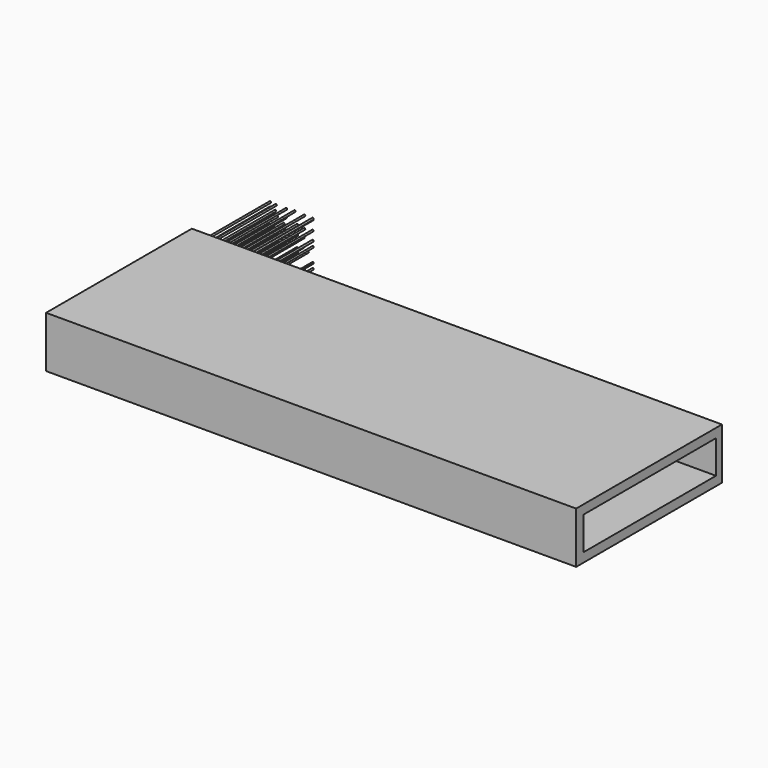
from build123d import *

# Parameters (mm, degrees)
F0_W     = 16
F0_H     = 5.5
F1_DEPTH = 1.55
F2_W     = 5
F2_H     = 1
F3_DEPTH = 5
F5_R     = 0.025
F6_DEPTH = 2.5


# Not quite as in the source:
# - ends of sketch curves that miss each other by under 0.0002 mm in the source are joined


with BuildPart() as f1:
    # F0 (on Top) → F1 (new body)
    with BuildSketch(Plane.XY):
        with Locations((-47.4078631294, 31.0802683234)):
            Rectangle(F0_W, F0_H)
    extrude(amount=F1_DEPTH)

    # F2 (on face) → F3 (cut)
    with BuildSketch(Plane.YZ.offset(-39.4078631294)):
        with Locations((31.1061264947, 0.7766577088)):
            Rectangle(F2_W, F2_H)
    extrude(amount=-F3_DEPTH, mode=Mode.SUBTRACT)

    # F5 (on face) → F6 (join)
    with BuildSketch(Plane(origin=(0, 33.8302683234, 0), x_dir=(-1, 0, 0), z_dir=(0, 1, 0))):
        with Locations((54.8700392246, 1.3386292849)):
            Circle(F5_R)
        with Locations((54.8874177039, 1.1790156132)):
            Circle(F5_R)
        with Locations((55.0432913005, 1.0209160391)):
            Circle(F5_R)
        with Locations((55.0438500941, 1.2124801287)):
            Circle(F5_R)
        with Locations((54.8334904015, 1.0420758044)):
            Circle(F5_R)
        with Locations((54.9310669303, 0.7820026949)):
            Circle(F5_R)
        with Locations((55.0913289189, 0.7783339825)):
            Circle(F5_R)
        with Locations((54.2229190469, 0.5845874548)):
            Circle(F5_R)
        with Locations((54.5544400811, 0.7645821315)):
            Circle(F5_R)
        with Locations((54.636053741, 0.9168148972)):
            Circle(F5_R)
        with Locations((54.5544400811, 1.1157006957)):
            Circle(F5_R)
        with Locations((55.2944801748, 0.2964735031)):
            Circle(F5_R)
        with Locations((55.104508996, 0.3338116512)):
            Circle(F5_R)
        with Locations((53.7547841668, 0.5845874548)):
            Circle(F5_R)
        with BuildLine():
            ThreePointArc((53.7297844731, 0.1600140822), (53.7547222964, 0.1351379083), (53.7797829418, 0.1598903449))
            ThreePointArc((53.7797829418, 0.1598903449), (53.7797838606, 0.1600140868), (53.7797841668, 0.1601378317))
            ThreePointArc((53.7797841668, 0.1601378317), (53.7547222964, 0.1848902562), (53.7297844731, 0.1600140822))
        make_face()
        with Locations((54.8100434244, 0.1598903327)):
            Circle(F5_R)
        with Locations((55.104508996, 0.1598903327)):
            Circle(F5_R)
        with Locations((55.104508996, 0.4052986042)):
            Circle(F5_R)
        with Locations((54.8100434244, 0.3365922312)):
            Circle(F5_R)
        with Locations((54.9537017941, 0.4052986042)):
            Circle(F5_R)
        with Locations((54.2229190469, 0.7517706254)):
            Circle(F5_R)
        with Locations((54.3024428189, 1.3575049816)):
            Circle(F5_R)
        with Locations((54.9545623362, 0.2160392905)):
            Circle(F5_R)
        with Locations((54.5537918806, 0.38031445)):
            Circle(F5_R)
        with BuildLine():
            Line((53.7297841668, 0), (53.7797841668, 0))
            ThreePointArc((53.7797841668, 0), (53.7547841668, 0.025), (53.7297841668, 0))
        make_face()
        with BuildLine():
            ThreePointArc((53.7297841668, 0), (53.7547841668, -0.025), (53.7797841668, 0))
            Line((53.7797841668, 0), (53.7297841668, 0))
        make_face()
        with Locations((54.2229190469, 0.2990950306)):
            Circle(F5_R)
        with Locations((54.5537918806, 1.3386292849)):
            Circle(F5_R)
        with BuildLine():
            ThreePointArc((53.7300307947, 0.7482676883), (53.7530283626, 0.7198264845), (53.7797841668, 0.7447647513))
            ThreePointArc((53.7797841668, 0.7447647513), (53.7797224336, 0.7465205555), (53.7795375389, 0.7482676883))
            ThreePointArc((53.7795375389, 0.7482676883), (53.7547841668, 0.7267706254), (53.7300307947, 0.7482676883))
        make_face()
        with BuildLine():
            ThreePointArc((53.7300307947, 0.7482676883), (53.7547841668, 0.7267706254), (53.7795375389, 0.7482676883))
            ThreePointArc((53.7795375389, 0.7482676883), (53.7547841668, 0.7697647513), (53.7300307947, 0.7482676883))
        make_face()
        with BuildLine():
            ThreePointArc((53.7300307947, 0.7482676883), (53.7547841668, 0.7697647513), (53.7795375389, 0.7482676883))
            ThreePointArc((53.7795375389, 0.7482676883), (53.7797224336, 0.7500148212), (53.7797841668, 0.7517706254))
            ThreePointArc((53.7797841668, 0.7517706254), (53.7530283626, 0.7767088922), (53.7300307947, 0.7482676883))
        make_face()
        with BuildLine():
            ThreePointArc((54.244569682, 0.39281445), (54.2470671925, 0.3988439739), (54.2479190469, 0.40531445))
            ThreePointArc((54.2479190469, 0.40531445), (54.2164485708, 0.4294625957), (54.2012684118, 0.39281445))
            ThreePointArc((54.2012684118, 0.39281445), (54.2229190469, 0.40531445), (54.244569682, 0.39281445))
        make_face()
        with BuildLine():
            ThreePointArc((54.244569682, 0.39281445), (54.2229190469, 0.40531445), (54.2012684118, 0.39281445))
            ThreePointArc((54.2012684118, 0.39281445), (54.2229190469, 0.38031445), (54.244569682, 0.39281445))
        make_face()
        with BuildLine():
            ThreePointArc((54.244569682, 0.39281445), (54.2229190469, 0.38031445), (54.2012684118, 0.39281445))
            ThreePointArc((54.2012684118, 0.39281445), (54.2164485708, 0.3561663044), (54.2479190469, 0.38031445))
            ThreePointArc((54.2479190469, 0.38031445), (54.2470671925, 0.3867849261), (54.244569682, 0.39281445))
        make_face()
        with BuildLine():
            ThreePointArc((53.7778465192, 1.328979005), (53.7792949686, 1.3337078425), (53.7797841668, 1.3386292849))
            ThreePointArc((53.7797841668, 1.3386292849), (53.74679086, 1.3623169831), (53.7348956031, 1.3234818418))
            ThreePointArc((53.7348956031, 1.3234818418), (53.7547841668, 1.3386292849), (53.7778465192, 1.328979005))
        make_face()
        with BuildLine():
            ThreePointArc((53.7778465192, 1.328979005), (53.7547841668, 1.3386292849), (53.7348956031, 1.3234818418))
            ThreePointArc((53.7348956031, 1.3234818418), (53.7579579555, 1.3138315619), (53.7778465192, 1.328979005))
        make_face()
        with BuildLine():
            ThreePointArc((53.7778465192, 1.328979005), (53.7579579555, 1.3138315619), (53.7348956031, 1.3234818418))
            ThreePointArc((53.7348956031, 1.3234818418), (53.7530365131, 1.2893207601), (53.7829579555, 1.3138315619))
            ThreePointArc((53.7829579555, 1.3138315619), (53.7816456537, 1.3218248687), (53.7778465192, 1.328979005))
        make_face()
        with Locations((54.0354177356, 0.7447647513)):
            Circle(F5_R)
        with Locations((53.9033412933, 0.4030845012)):
            Circle(F5_R)
        with Locations((54.2229190469, 1.0209160391)):
            Circle(F5_R)
        with Locations((54.0087483823, 0.9824559093)):
            Circle(F5_R)
        with Locations((53.7547841668, 1.0209160391)):
            Circle(F5_R)
        with Locations((55.0438500941, 1.3575049816)):
            Circle(F5_R)
        with Locations((55.0438500941, 0.5675284774)):
            Circle(F5_R)
        with Locations((54.237511009, 0.1731978846)):
            Circle(F5_R)
        with Locations((54.0354177356, 0.4944094107)):
            Circle(F5_R)
        with Locations((54.0087483823, 1.3386292849)):
            Circle(F5_R)
    extrude(amount=F6_DEPTH)


solid = f1.part
